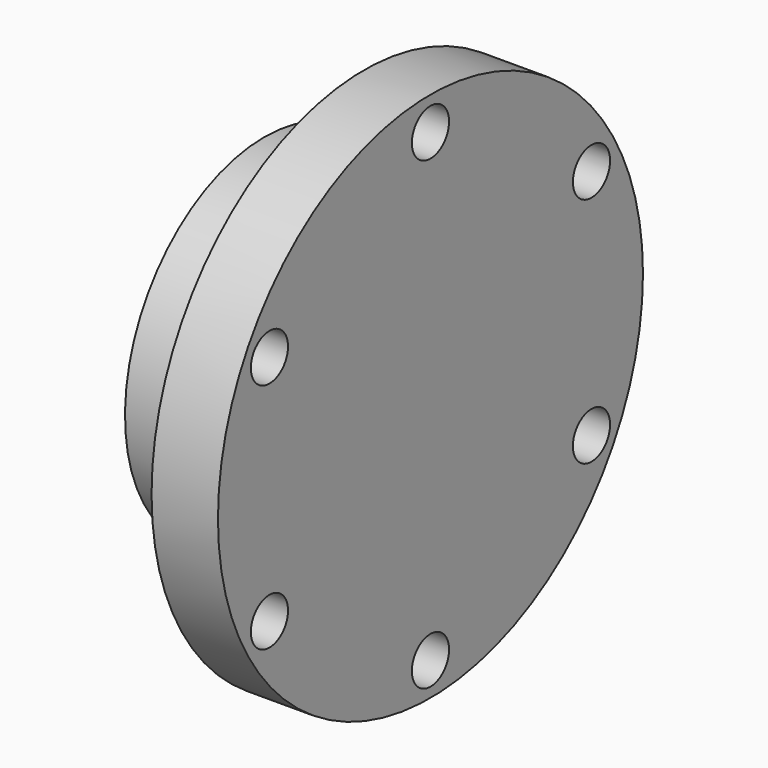
from build123d import *

# Parameters (mm, degrees)
F0_W            = 15
F0_H            = 26.25
F2_R            = 40
F2_R_2          = 26.25
F3_DEPTH        = 10
F4_R            = 3.5
F5_DEPTH        = 25.001
F5_COPIES_COUNT = 6


# Not quite as in the source:
# - a pattern or mirror of a feature is missing from the dataset's text; its kind, count and spacing are read off the source's solid


with BuildPart() as f1:
    # F0 (on Front) → F1 (revolve)
    with BuildSketch(Plane.XZ):
        with Locations((7.5, 13.125)):
            Rectangle(F0_W, F0_H)
    revolve(axis=Axis((-28.7704151153, 0, 0), (-1, 0, 0)))

    # F2 (on face) → F3 (join)
    with BuildSketch(Plane.YZ.offset(15)):
        Circle(F2_R)
        Circle(F2_R_2, mode=Mode.SUBTRACT)
        Circle(F2_R_2)
    extrude(amount=F3_DEPTH)

    # F4 (on face) → F5 (cut, through all)
    with BuildSketch(Plane(origin=(0, 0, 0), x_dir=(0, -1, 0), z_dir=(-1, 0, 0))):
        with Locations((30.3108891325, 17.5)):
            Circle(F4_R)
    f5 = extrude(amount=-F5_DEPTH, mode=Mode.SUBTRACT)

    # F5_copies: F5 ×6 about axis
    f5_copies_axis = Axis((0, 0, 0), (1, 0, 0))
    for i in range(1, F5_COPIES_COUNT):
        add(f5.rotate(f5_copies_axis, i * 360 / F5_COPIES_COUNT), mode=Mode.SUBTRACT)


solid = f1.part
